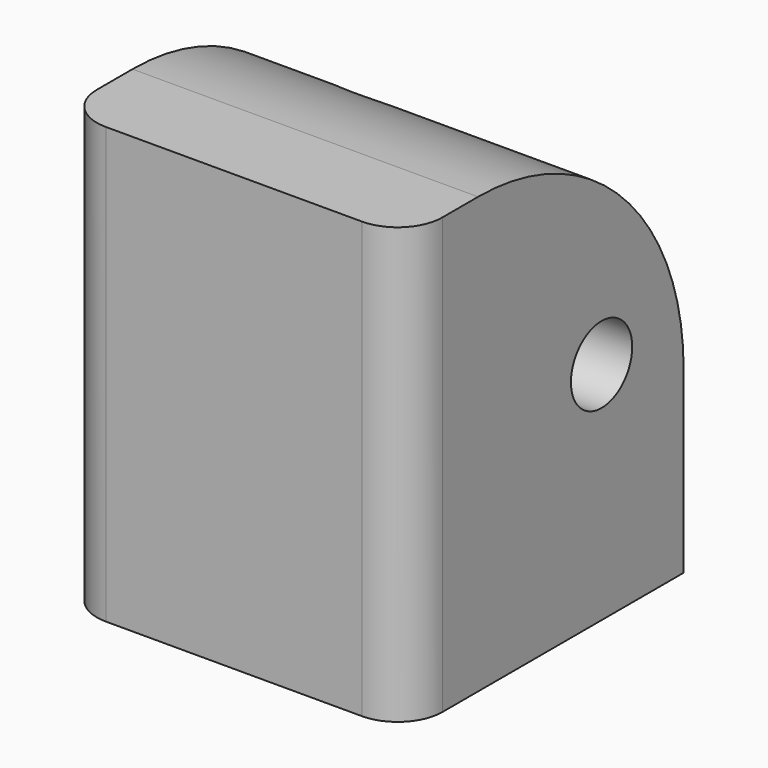
from build123d import *

# Parameters (mm, degrees)
F0_R        = 6.5
F1_DEPTH    = 63
F2_T1_DEPTH = 235.8944443027
F3_R        = 5.5443537003
F4_DEPTH    = 50.0010001


# Not quite as in the source:
# - a fillet or chamfer that OpenCascade refuses, or shapes differently, is made with other operations: its cross-section is extruded or revolved along the edge and cut away or added


with BuildPart() as f1:
    # F0 (on Top) → F1 (new body)
    with BuildSketch(Plane.XY):
        with BuildLine():
            ThreePointArc((-25, -18.57671062), (-23.1040174372, -23.1540174372), (-18.52671062, -25.05))
            Line((-18.52671062, -25.05), (18.52671062, -25.05))
            ThreePointArc((18.52671062, -25.05), (23.1040174372, -23.1540174372), (25, -18.57671062))
            Line((25, -18.57671062), (25, 25.05))
            Line((25, 25.05), (-25, 25.05))
            Line((-25, 25.05), (-25, -18.57671062))
        make_face()
        with Locations((-7.6206641026, 13.05)):
            Circle(F0_R, mode=Mode.SUBTRACT)
    extrude(amount=F1_DEPTH)

    # F2: fillet of radius 37.1788888605 on 1 edges, made by hand

    # F2_s2 → F2_t1 (cut)
    with BuildSketch(Plane.YZ.offset(-117.9472221514)):
        with BuildLine():
            ThreePointArc((25.05, 25.8211111395), (14.1605555697, 52.1105555697), (-12.1288888605, 63))
            Line((-12.1288888605, 63), (25.05, 63))
            Line((25.05, 63), (25.05, 25.8211111395))
        make_face()
    extrude(amount=F2_T1_DEPTH, mode=Mode.SUBTRACT)

    # F3 (on face) → F4 (cut, through all)
    with BuildSketch(Plane.YZ.offset(25)):
        with Locations((10.2042127401, 32.5643420219)):
            Circle(F3_R)
    extrude(amount=-F4_DEPTH, mode=Mode.SUBTRACT)


solid = f1.part
